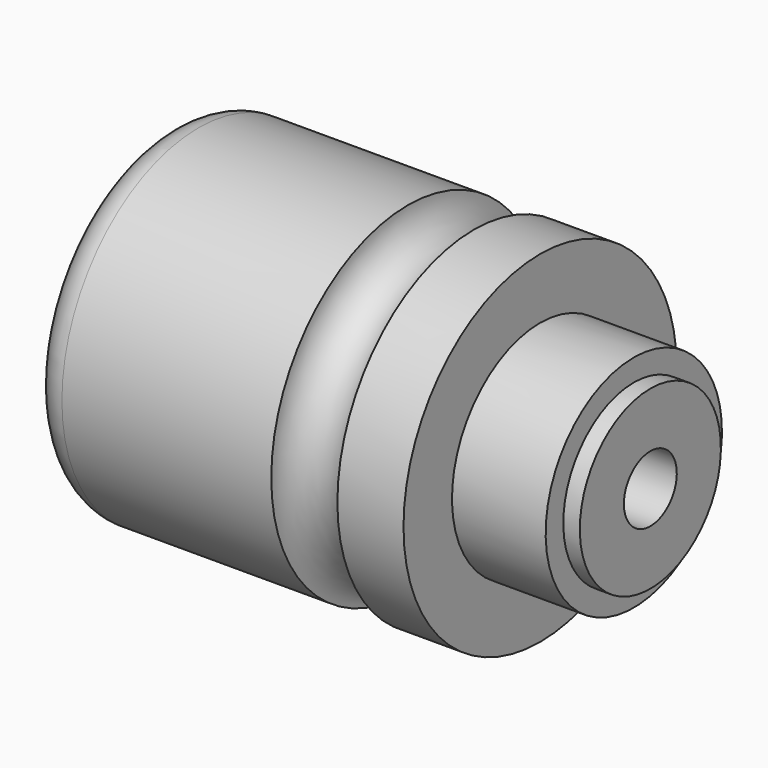
from build123d import *

# Parameters (mm, degrees)
F4_R = 5.99999


# Not quite as in the source:
# - a fillet or chamfer is up to 0.001 mm smaller than in the source, because OpenCascade refuses the exact size


with BuildPart() as f1:
    # F0 (on Front) → F1 (revolve)
    with BuildSketch(Plane.XZ):
        with BuildLine():
            Line((0, 31), (0, 0))
            Line((0, 0), (88, 0))
            Line((88, 0), (88, 16))
            Line((88, 16), (85, 16))
            Line((85, 16), (85, 20))
            Line((85, 20), (68, 20))
            Line((68, 20), (68, 31))
            Line((68, 31), (56, 31))
            ThreePointArc((56, 31), (50, 25), (44, 31))
            Line((44, 31), (0, 31))
        make_face()
    revolve(axis=Axis((44, 0, 0), (-1, 0, 0)))

    # F2 (on Front) → F3 (revolve, cut)
    with BuildSketch(Plane.XZ):
        Polygon((0, 25), (0, 0), (88, 0), (88, 6), (30, 6), (30, 16), (22, 16), (22, 20.5), (15, 20.5), (15, 12.5), (12, 12.5), (12, 16), (1.5, 16), (1.5, 25), align=None)
    revolve(axis=Axis((-15.3110799765, 0, 0), (-1, 0, 0)), mode=Mode.SUBTRACT)

    # F4 (radius 6 in the source; OpenCascade refuses exactly that, so slightly less here)
    f4_edges = [f1.edges().sort_by_distance(p)[0] for p in [
        (0, 0, -31),
    ]]
    fillet(f4_edges, radius=F4_R)


solid = f1.part
